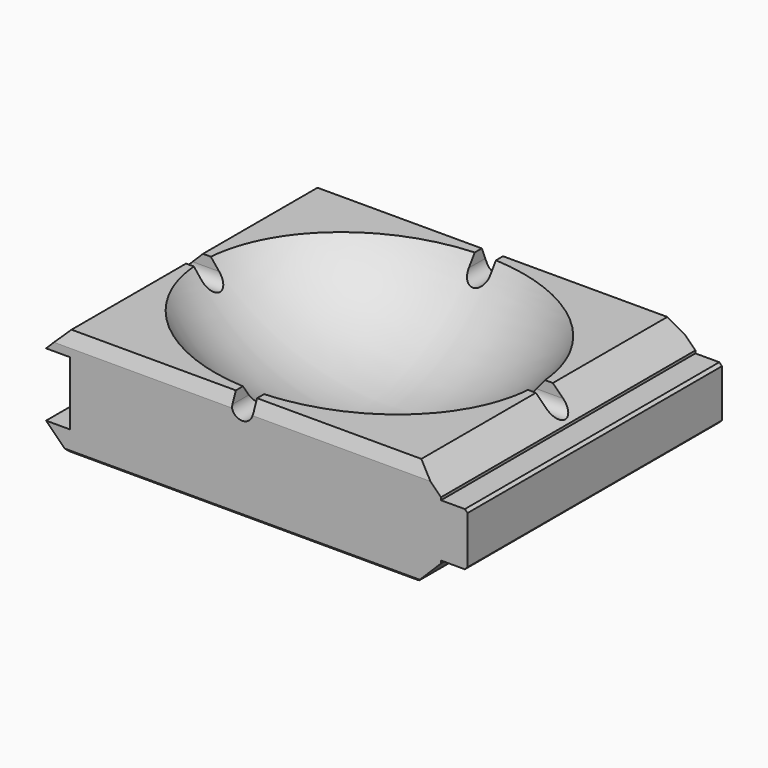
from build123d import *

# Parameters (mm, degrees)
F1_DEPTH    = 120
F2_SIZE2    = 2
F2_SIZE     = 5
F2_2_SIZE2  = 2
F2_2_SIZE   = 5
F3_T1_DEPTH = 162.2902937834
F3_T3_DEPTH = 166.2902937834
F4_T1_DEPTH = 125.1433659759
F4_T3_DEPTH = 137.1433659759
F4_T5_DEPTH = 122.2571417204
F10_DEPTH   = 120.001
F12_DEPTH   = 159.001


# Not quite as in the source:
# - a fillet or chamfer that OpenCascade refuses, or shapes differently, is made with other operations: its cross-section is extruded or revolved along the edge and cut away or added


with BuildPart() as f1:
    # F0 (on Front) → F1 (new body)
    with BuildSketch(Plane.XZ):
        Polygon((-75, 8), (-75, 0), (75, 0), (75, 10), (85, 10), (85, 30), (75, 30), (75, 40), (-75, 40), (-75, 32), (-65, 32), (-65, 8), align=None)
    extrude(amount=-F1_DEPTH)

    # F2
    f2_edges = [f1.edges().sort_by_distance(p)[0] for p in [
        (0, 0, 40),
    ]]
    f2_side = f1.faces().sort_by_distance((5.503356, 0, 20))[0]
    chamfer(f2_edges, length=F2_SIZE, length2=F2_SIZE2, reference=f2_side)

    # F2#2
    f2_2_edges = [f1.edges().sort_by_distance(p)[0] for p in [
        (0, 120, 40),
    ]]
    f2_2_side = f1.faces().sort_by_distance((5.503356, 120, 20))[0]
    chamfer(f2_2_edges, length=F2_2_SIZE, length2=F2_2_SIZE2, reference=f2_2_side)

    # F3: chamfer of 9 on 4 edges, made by hand

    # F3_s2 → F3_t1 (cut)
    with BuildSketch(Plane.XZ.offset(-141.1451468917)):
        Polygon((75, 31), (66, 40), (75, 40), align=None)
        Polygon((-66, 40), (-75, 31), (-75, 40), align=None)
    extrude(amount=F3_T1_DEPTH, mode=Mode.SUBTRACT)

    # F3_s4 → F3_t3 (cut)
    with BuildSketch(Plane.XZ.offset(-143.1451468917)):
        Polygon((-66, 0), (-75, 9), (-75, 0), align=None)
        Polygon((75, 9), (66, 0), (75, 0), align=None)
    extrude(amount=F3_T3_DEPTH, mode=Mode.SUBTRACT)

    # F4: chamfer of 1 on 6 edges, made by hand

    # F4_s2 → F4_t1 (cut)
    with BuildSketch(Plane.XZ.offset(-122.571682988)):
        Polygon((84, 30), (85, 29), (85, 30), align=None)
        Polygon((85, 11), (84, 10), (85, 10), align=None)
    extrude(amount=F4_T1_DEPTH, mode=Mode.SUBTRACT)

    # F4_s4 → F4_t3 (cut)
    with BuildSketch(Plane.YZ.offset(-68.571682988)):
        Polygon((0, 1), (1, 0), (0, 0), align=None)
        Polygon((120, 1), (119, 0), (120, 0), align=None)
    extrude(amount=F4_T3_DEPTH, mode=Mode.SUBTRACT)

    # F4_s6 → F4_t5 (cut)
    with BuildSketch(Plane.XZ.offset(-121.1285708602)):
        Polygon((-65.5857864376, 0), (-66.2928932188, 0.2928932188), (-66, 0), align=None)
        Polygon((66.2928932188, 0.2928932188), (65.5857864376, 0), (66, 0), align=None)
    extrude(amount=F4_T5_DEPTH, mode=Mode.SUBTRACT)

    # F6 (on offset) → F8 (revolve, cut)
    with BuildSketch(Plane.XY.offset(75)):
        with BuildLine():
            Line((-75, 60), (75, 60))
            add(Edge.make_bspline(
                [(75, 60), (75, 125), (0, 125), (-75, 125), (-75, 60)],
                knots=[0, 0, 0, 1.5707963268, 1.5707963268, 3.1415926536, 3.1415926536, 3.1415926536], degree=2, weights=[1, 0.7071067812, 1, 0.7071067812, 1]))
        make_face()
    revolve(axis=Axis((-0.8174791932, 60, 75), (1, 0, 0)), mode=Mode.SUBTRACT)

    # F9 (on face) → F10 (cut, through all)
    with BuildSketch(Plane.XZ):
        with BuildLine():
            Line((4, 36), (4, 40))
            Line((4, 40), (-4, 40))
            Line((-4, 40), (-4, 36))
            ThreePointArc((-4, 36), (0, 32), (4, 36))
        make_face()
    extrude(amount=-F10_DEPTH, mode=Mode.SUBTRACT)

    # F11 (on face) → F12 (cut, through all)
    with BuildSketch(Plane.YZ.offset(85)):
        with BuildLine():
            Line((64, 36.1), (64, 40))
            Line((64, 40), (56, 40))
            Line((56, 40), (56, 36.1))
            ThreePointArc((56, 36.1), (60, 32.1), (64, 36.1))
        make_face()
    extrude(amount=-F12_DEPTH, mode=Mode.SUBTRACT)


solid = f1.part
